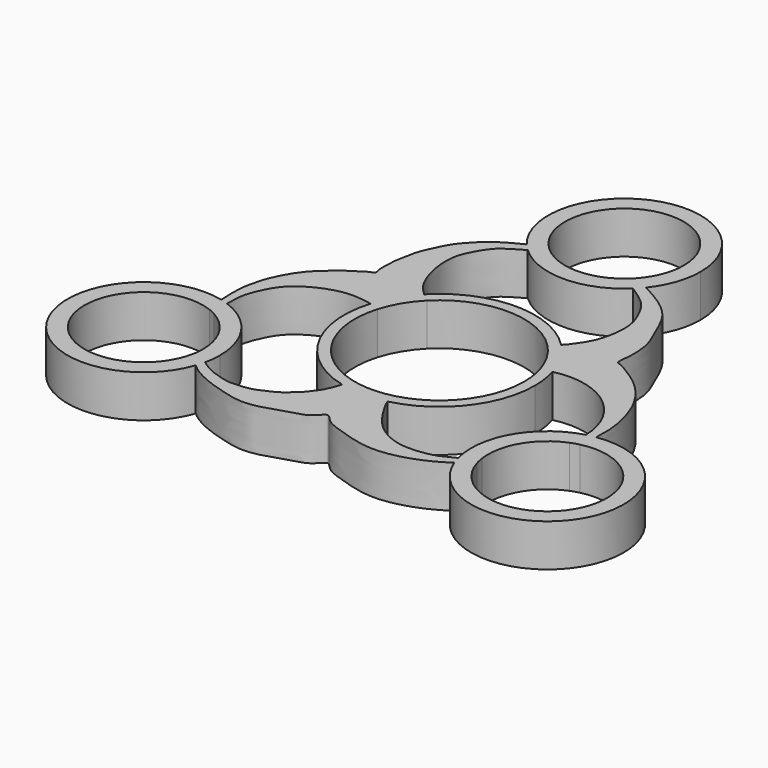
from build123d import *

# Parameters (mm, degrees)
F1_DEPTH = 6.35


with BuildPart() as f1:
    # F0 (on Top) → F1 (new body)
    with BuildSketch(Plane.XY):
        with BuildLine():
            ThreePointArc((12.1979827597, 3.535423114), (12.5738693537, 1.7854437757), (12.7, 0))
            ThreePointArc((12.7, 0), (10.0261967093, -7.79521517), (3.1306488904, -12.3080882969))
            add(Edge.make_bspline(
                [(3.363740595, -13.9083727332), (3.2442211047, -13.5834802382), (3.0616730097, -12.9484213085), (3.1089422782, -12.5172223169), (3.1306488904, -12.3080882969)],
                knots=[0.9737577336, 0.9737577336, 0.9737577336, 0.9737577336, 0.9873943893, 1, 1, 1, 1], degree=3))
            ThreePointArc((3.363740595, -13.9083727332), (11.2447884463, -8.8494245957), (14.309352986, 0))
            ThreePointArc((14.309352986, 0), (14.1647786053, 2.0289479883), (13.7339768745, 4.016897072))
            ThreePointArc((13.7339768745, 4.016897072), (12.9568547986, 3.8052706492), (12.1979827597, 3.535423114))
        make_face()
        with BuildLine():
            ThreePointArc((9.0393838541, 8.9207364908), (10.954763129, 6.4251976457), (12.1979827597, 3.535423114))
            ThreePointArc((12.1979827597, 3.535423114), (12.9568547986, 3.8052706492), (13.7339768745, 4.016897072))
            ThreePointArc((13.7339768745, 4.016897072), (12.356609853, 7.2160775923), (10.2471131468, 9.9877051935))
            add(Edge.make_bspline(
                [(10.2471131468, 9.9877051935), (9.9232107522, 9.6798780377), (9.351132595, 9.2068135599), (9.1315325532, 9.0053976698), (9.0393838541, 8.9207364908)],
                knots=[0.9630977835, 0.9630977835, 0.9630977835, 0.9630977835, 0.9846295847, 1, 1, 1, 1], degree=3))
        make_face()
        with BuildLine():
            add(Edge.make_bspline(
                [(3.363740595, -13.9083727332), (3.2442211047, -13.5834802382), (3.0616730097, -12.9484213085), (3.1089422782, -12.5172223169), (3.1306488904, -12.3080882969)],
                knots=[0.9737577336, 0.9737577336, 0.9737577336, 0.9737577336, 0.9873943893, 1, 1, 1, 1], degree=3))
            ThreePointArc((3.1306488904, -12.3080882969), (-0.0390202402, -12.6999400558), (-3.2062216412, -12.2886184247))
            add(Edge.make_bspline(
                [(-3.2062216412, -12.2886184247), (-3.2435862999, -12.7247349168), (-3.2885775207, -13.2545873407), (-3.4299574494, -13.7893304451), (-3.4577927192, -13.8852890639)],
                knots=[0, 0, 0, 0, 0.0176926318, 0.0215554453, 0.0215554453, 0.0215554453, 0.0215554453], degree=3))
            ThreePointArc((-3.4577927192, -13.8852890639), (-0.0484217354, -14.309271058), (3.363740595, -13.9083727332))
        make_face()
        with BuildLine():
            ThreePointArc((-9.0313311184, 8.9288889695), (0.005729517, 12.6999987076), (9.0393838541, 8.9207364908))
            add(Edge.make_bspline(
                [(10.2471131468, 9.9877051935), (9.9232107522, 9.6798780377), (9.351132595, 9.2068135599), (9.1315325532, 9.0053976698), (9.0393838541, 8.9207364908)],
                knots=[0.9630977835, 0.9630977835, 0.9630977835, 0.9630977835, 0.9846295847, 1, 1, 1, 1], degree=3))
            ThreePointArc((10.2471131468, 9.9877051935), (-0.0109633608, 14.3093487861), (-10.2624056216, 9.9719914628))
            add(Edge.make_bspline(
                [(-9.0313311184, 8.9288889695), (-9.4487098634, 9.2705061134), (-9.8662421937, 9.6122685884), (-10.2624056216, 9.9719914628)],
                knots=[0, 0, 0, 0, 0.0111174301, 0.0111174301, 0.0111174301, 0.0111174301], degree=3))
        make_face()
        with BuildLine():
            ThreePointArc((10.2471131468, 9.9877051935), (12.356609853, 7.2160775923), (13.7339768745, 4.016897072))
            ThreePointArc((13.7339768745, 4.016897072), (22.6213268762, 2.0857346054), (26.7638742582, -6.0107880872))
            ThreePointArc((26.7638742582, -6.0107880872), (27.4125460464, -5.8521775606), (28.0693734163, -5.7317192929))
            add(Edge.make_bspline(
                [(28.0693734163, -5.7317192928), (28.0908448663, -5.3731517648), (28.1861747627, -3.0109562541), (27.749558093, -0.5133237083), (26.6719185003, 2.9301219991), (25.4157041022, 4.8818668184), (25.0606077232, 5.4096449257), (23.1974632753, 7.8967221343), (18.7843205423, 10.5309990469), (18.0312497954, 10.5798070842), (18.3811975836, 12.6295870836), (18.335387886, 16.2496050809), (16.6672868668, 19.632117318), (15.0493924505, 23.6629486703), (11.9963770049, 25.9005801835), (9.3079958484, 27.3351514106), (8.9392781783, 27.5237386375)],
                knots=[0.0686911974, 0.0686911974, 0.0686911974, 0.0686911974, 0.0770625743, 0.1250692546, 0.1682015773, 0.2016986428, 0.2192050888, 0.2596345178, 0.3116854663, 0.3277616325, 0.357626719, 0.4018708944, 0.4463436454, 0.4924730526, 0.5489378858, 0.5577650476, 0.5577650476, 0.5577650476, 0.5577650476], degree=3))
            ThreePointArc((8.9392781783, 27.5237386375), (8.4361841281, 26.9344845866), (7.8943251244, 26.3806680284))
            add(Edge.make_bspline(
                [(7.8943251244, 26.3806680284), (8.4148020655, 26.072489779), (9.8207087272, 25.0972655112), (11.4008317967, 23.8393962796), (12.7154437587, 21.3058333832), (13.4643703621, 19.2153114545), (13.487767982, 16.5541309423), (12.7738805207, 13.4867000838), (11.6527838604, 11.777088674), (10.936534424, 10.6698737269), (10.366109532, 10.1007958017), (10.2471131468, 9.9877051935)],
                knots=[0.6848165544, 0.6848165544, 0.6848165544, 0.6848165544, 0.7057956752, 0.7426414418, 0.7804706255, 0.8144755937, 0.8516859329, 0.8922387418, 0.9247476761, 0.9551873556, 0.9630977835, 0.9630977835, 0.9630977835, 0.9630977835], degree=3))
        make_face()
        with BuildLine():
            add(Edge.make_bspline(
                [(-3.2062216412, -12.2886184247), (-3.2435862999, -12.7247349168), (-3.2885775207, -13.2545873407), (-3.4299574494, -13.7893304451), (-3.4577927192, -13.8852890639)],
                knots=[0, 0, 0, 0, 0.0176926318, 0.0215554453, 0.0215554453, 0.0215554453, 0.0215554453], degree=3))
            ThreePointArc((-3.2062216412, -12.2886184247), (-11.0679306792, -6.228234941), (-12.1680586093, 3.6370798286))
            add(Edge.make_bspline(
                [(-13.6805620316, 4.1952121968), (-13.4436838321, 4.1415517594), (-12.7953614065, 3.9690441824), (-12.4205580368, 3.769996542), (-12.1680586093, 3.6370798286)],
                knots=[0.9804169862, 0.9804169862, 0.9804169862, 0.9804169862, 0.9869875731, 1, 1, 1, 1], degree=3))
            ThreePointArc((-13.6805620316, 4.1952121968), (-12.4562005584, -7.0427729288), (-3.4577927192, -13.8852890639))
        make_face()
        with BuildLine():
            add(Edge.make_bspline(
                [(18.7441266975, -19.9228869496), (18.0486010574, -20.282431647), (16.5041031929, -21.1337661556), (14.3497934766, -21.5215057085), (11.2348222617, -21.7472578966), (7.8237393097, -20.2593616193), (5.6360308604, -18.0063979855), (4.1304020556, -15.5442912857), (3.5977305956, -14.5157527694), (3.3928512144, -13.9875047789), (3.363740595, -13.9083727332)],
                knots=[0.7955891005, 0.7955891005, 0.7955891005, 0.7955891005, 0.8189494254, 0.841960922, 0.8688237268, 0.8981267776, 0.9256229436, 0.9515003665, 0.9704363381, 0.9737577336, 0.9737577336, 0.9737577336, 0.9737577336], degree=3))
            ThreePointArc((3.363740595, -13.9083727332), (-0.0484217354, -14.309271058), (-3.4577927192, -13.8852890639))
            add(Edge.make_bspline(
                [(-3.4577927192, -13.8852890639), (-3.56467622, -14.2537565951), (-3.8875885257, -15.0858670187), (-4.395377985, -16.3369768283), (-5.1592727376, -17.2342121704), (-5.8768462607, -18.2950992181), (-6.9156654614, -19.1057392203), (-7.9469878233, -20.0471955678), (-9.1177528934, -20.5439332885), (-10.4408920068, -21.2379911781), (-11.9275421158, -21.5685916523), (-13.3895555039, -21.6459776552), (-13.8617944711, -21.6400506083), (-14.3017979669, -21.7027035652), (-17.183723559, -21.0200808639), (-18.7684540581, -20.0590219662), (-19.5179344331, -19.4775341217)],
                knots=[0.0215554453, 0.0215554453, 0.0215554453, 0.0215554453, 0.0363881028, 0.0548777285, 0.0715243999, 0.0887731028, 0.1064890588, 0.1245483308, 0.1418573875, 0.1605160383, 0.179942663, 0.1984165029, 0.2084162614, 0.2180022527, 0.2438992002, 0.2696875695, 0.2696875695, 0.2696875695, 0.2696875695], degree=3))
            ThreePointArc((-19.5179344331, -19.4775341217), (-19.6842633145, -20.140683936), (-19.8899435093, -20.7927028242))
            add(Edge.make_bspline(
                [(-19.8899435093, -20.7927028242), (-19.5053999908, -21.1412232423), (-18.421181972, -21.9802458066), (-16.0493936535, -23.1187044109), (-14.0030480662, -23.7091152957), (-9.4186989056, -25.2065289459), (-4.4872481249, -23.2076928696), (-1.3008667338, -22.5759404404), (-0.0119091358, -20.3631569563), (1.1345603492, -22.2720709759), (3.8195402322, -23.1392079338), (7.6272449858, -24.42130256), (11.7818612833, -24.4535976361), (16.3095086913, -22.95262019), (18.294497797, -21.702246116), (19.1372684615, -21.1419244632)],
                knots=[0.3583161785, 0.3583161785, 0.3583161785, 0.3583161785, 0.3741552252, 0.4000090879, 0.4227597006, 0.4556567182, 0.4912178975, 0.5190290749, 0.5393412725, 0.5581268934, 0.5841470097, 0.6149491691, 0.6463952944, 0.6807440143, 0.7044884009, 0.7044884009, 0.7044884009, 0.7044884009], degree=3))
            ThreePointArc((19.1372684615, -21.1419244632), (18.9236082439, -20.5379170475), (18.7441266975, -19.9228869496))
        make_face()
        with BuildLine():
            ThreePointArc((-12.1680586093, 3.6370798286), (-10.9249412906, 6.475774687), (-9.0313311184, 8.9288889695))
            add(Edge.make_bspline(
                [(-9.0313311184, 8.9288889695), (-9.4487098634, 9.2705061134), (-9.8662421937, 9.6122685884), (-10.2624056216, 9.9719914628)],
                knots=[0, 0, 0, 0, 0.0111174301, 0.0111174301, 0.0111174301, 0.0111174301], degree=3))
            ThreePointArc((-10.2624056216, 9.9719914628), (-12.3149997841, 7.2868623696), (-13.6805620316, 4.1952121968))
            add(Edge.make_bspline(
                [(-13.6805620316, 4.1952121968), (-13.4436838321, 4.1415517594), (-12.7953614065, 3.9690441824), (-12.4205580368, 3.769996542), (-12.1680586093, 3.6370798286)],
                knots=[0.9804169862, 0.9804169862, 0.9804169862, 0.9804169862, 0.9869875731, 1, 1, 1, 1], degree=3))
        make_face()
        with BuildLine():
            ThreePointArc((28.0693734163, -5.7317192929), (27.4125460464, -5.8521775606), (26.7638742582, -6.0107880872))
            ThreePointArc((26.7638742582, -6.0107880872), (26.7154514397, -7.4054133304), (26.4847933941, -8.7816840901))
            ThreePointArc((26.4847933941, -8.7816840901), (27.1211091404, -8.5534785531), (27.7729255559, -8.3742835288))
            add(Edge.make_bspline(
                [(27.7729255559, -8.3742835288), (27.9153636471, -7.5821879417), (28.0154450564, -6.6323086159), (28.0693734163, -5.7317192928)],
                knots=[0.0476653874, 0.0476653874, 0.0476653874, 0.0476653874, 0.0686911974, 0.0686911974, 0.0686911974, 0.0686911974], degree=3))
        make_face()
        with BuildLine():
            ThreePointArc((26.4847933941, -8.7816840901), (26.7154514397, -7.4054133304), (26.7638742582, -6.0107880872))
            ThreePointArc((26.7638742582, -6.0107880872), (19.8993963954, -11.3212767476), (18.7441266975, -19.9228869496))
            add(Edge.make_bspline(
                [(21.0074985339, -18.3299627331), (20.8758294418, -18.4776732411), (20.2330176684, -19.2024066572), (19.4784607209, -19.5448948869), (18.7861304092, -19.9011735706), (18.7441266975, -19.9228869496)],
                knots=[0.7662125489, 0.7662125489, 0.7662125489, 0.7662125489, 0.7721682582, 0.7941783396, 0.7955891005, 0.7955891005, 0.7955891005, 0.7955891005], degree=3))
            ThreePointArc((21.0074985339, -18.3299627331), (22.0905705657, -12.6061156205), (26.4847933941, -8.7816840901))
        make_face()
        with BuildLine():
            add(Edge.make_bspline(
                [(21.0074985339, -18.3299627331), (20.8758294418, -18.4776732411), (20.2330176684, -19.2024066572), (19.4784607209, -19.5448948869), (18.7861304092, -19.9011735706), (18.7441266975, -19.9228869496)],
                knots=[0.7662125489, 0.7662125489, 0.7662125489, 0.7662125489, 0.7721682582, 0.7941783396, 0.7955891005, 0.7955891005, 0.7955891005, 0.7955891005], degree=3))
            ThreePointArc((18.7441266975, -19.9228869496), (18.9236082439, -20.5379170475), (19.1372684615, -21.1419244632))
            add(Edge.make_bspline(
                [(19.1372684615, -21.1419244632), (19.375504243, -20.9835318275), (20.0960831119, -20.4976698432), (20.8777393147, -19.9759281537), (21.2980232313, -19.6212498212)],
                knots=[0.7044884009, 0.7044884009, 0.7044884009, 0.7044884009, 0.7112005027, 0.7245782298, 0.7245782298, 0.7245782298, 0.7245782298], degree=3))
            ThreePointArc((21.2980232313, -19.6212498212), (21.1286962311, -18.9810205461), (21.0074985339, -18.3299627331))
        make_face()
        with BuildLine():
            ThreePointArc((-13.6805620316, 4.1952121968), (-12.3149997841, 7.2868623696), (-10.2624056216, 9.9719914628))
            add(Edge.make_bspline(
                [(-10.2624056216, 9.9719914628), (-10.7762356065, 10.4385574962), (-12.0701262188, 11.7836146151), (-13.1133522735, 14.5988264438), (-13.5488715258, 16.8425720746), (-13.6112462054, 19.6390222529), (-12.6179615134, 21.8826004391), (-11.2252292617, 24.1374130376), (-9.9097624261, 25.0601310132), (-8.4142072138, 25.9632491001), (-7.8031976483, 26.2945871618)],
                knots=[0.0111174301, 0.0111174301, 0.0111174301, 0.0111174301, 0.0255369058, 0.0501589029, 0.0704799639, 0.0922653526, 0.1133436415, 0.1345486053, 0.1523387172, 0.1705841628, 0.1705841628, 0.1705841628, 0.1705841628], degree=3))
            ThreePointArc((-7.8031976483, 26.2945871618), (-8.3174588735, 26.8065858605), (-8.7981938428, 27.3501860486))
            add(Edge.make_bspline(
                [(-8.7981938428, 27.3501860486), (-9.3008746077, 27.1141698538), (-10.2648697648, 26.631366973), (-11.2205700524, 26.0765871705), (-12.5077872547, 25.2419913168), (-13.5878297754, 24.2642475313), (-14.8266948114, 22.9775900037), (-15.7640079059, 21.7857963953), (-16.3601601941, 20.5369041311), (-17.0170024392, 19.2950238203), (-17.6605076418, 17.6054504392), (-17.7666020566, 16.8660360184), (-17.9689277925, 15.8439929239), (-18.2780826486, 14.5541624619), (-18.3309003318, 12.8876446559), (-18.3467578229, 11.5218615298), (-17.9795074421, 10.6008301963), (-18.9501500085, 10.4173362769), (-19.6024758542, 9.85743987), (-20.7203525072, 9.2646019513), (-22.1224625096, 8.1909741441), (-23.6705510338, 6.8483154141), (-24.6220525536, 5.8773240915), (-25.4499207491, 4.7537323699), (-26.2162314301, 3.5206531279), (-26.8908201735, 2.0300349867), (-27.2712398353, 1.1575955517), (-27.7898644912, -0.8805960027), (-28.0072247707, -2.066957359), (-28.0597819575, -3.9941490782), (-27.9650258271, -5.6406480469), (-27.9447560089, -5.9324288341)],
                knots=[0.272936701, 0.272936701, 0.272936701, 0.272936701, 0.2887777021, 0.3031918976, 0.319418999, 0.3356933449, 0.3534827997, 0.3699338291, 0.3853607611, 0.4015194954, 0.4192285536, 0.4307941219, 0.4440313196, 0.4595101079, 0.4768532228, 0.4927431634, 0.504260623, 0.5158482459, 0.5283617488, 0.5431378455, 0.5610783945, 0.5802108476, 0.5957692543, 0.6112674735, 0.627599259, 0.6443127052, 0.6577531603, 0.676599654, 0.6913368875, 0.7144941722, 0.7197456255, 0.7197456255, 0.7197456255, 0.7197456255], degree=3))
            ThreePointArc((-27.9447560089, -5.9324288341), (-27.367786238, -6.0909132425), (-26.7999005537, -6.2793735135))
            add(Edge.make_bspline(
                [(-26.7999005537, -6.2793735135), (-26.8048058193, -5.9710391039), (-26.8002842833, -5.0183376748), (-26.6902560699, -3.3465727044), (-25.8799280703, -1.2809508318), (-24.4697637739, 1.4971779335), (-21.1641836673, 3.6006813244), (-17.9496805149, 4.6242605842), (-15.6583644342, 4.5471697783), (-14.1750226558, 4.3072232365), (-13.6805620316, 4.1952121968)],
                knots=[0.8240259196, 0.8240259196, 0.8240259196, 0.8240259196, 0.8330622341, 0.8517096932, 0.8714224213, 0.8946727522, 0.9209129012, 0.9452655147, 0.9667015134, 0.9804169862, 0.9804169862, 0.9804169862, 0.9804169862], degree=3))
        make_face()
        with BuildLine():
            ThreePointArc((-7.8031976483, 26.2945871618), (0.0626780115, 23.2167052828), (7.8943251244, 26.3806680284))
            add(Edge.make_bspline(
                [(5.0609472835, 27.3377091334), (5.4064251806, 27.2499397098), (6.293948707, 27.2199440502), (7.3427878567, 26.7072373271), (7.8943251244, 26.3806680284)],
                knots=[0.6434177254, 0.6434177254, 0.6434177254, 0.6434177254, 0.6625854696, 0.6848165544, 0.6848165544, 0.6848165544, 0.6848165544], degree=3))
            ThreePointArc((5.0609472835, 27.3377091334), (0.0211748238, 25.7565586475), (-5.0260726198, 27.3136830957))
            add(Edge.make_bspline(
                [(-7.8031976483, 26.2945871618), (-7.6884792357, 26.356796624), (-7.0896108618, 26.6725649375), (-6.4348697652, 26.9157154858), (-5.3178085882, 27.1302396322), (-5.0260726198, 27.3136830957)],
                knots=[0.1705841628, 0.1705841628, 0.1705841628, 0.1705841628, 0.174009786, 0.189308331, 0.2026657268, 0.2026657268, 0.2026657268, 0.2026657268], degree=3))
        make_face()
        with BuildLine():
            add(Edge.make_bspline(
                [(5.0609472835, 27.3377091334), (5.4064251806, 27.2499397098), (6.293948707, 27.2199440502), (7.3427878567, 26.7072373271), (7.8943251244, 26.3806680284)],
                knots=[0.6434177254, 0.6434177254, 0.6434177254, 0.6434177254, 0.6625854696, 0.6848165544, 0.6848165544, 0.6848165544, 0.6848165544], degree=3))
            ThreePointArc((7.8943251244, 26.3806680284), (8.4361841281, 26.9344845866), (8.9392781783, 27.5237386375))
            add(Edge.make_bspline(
                [(8.9392781783, 27.5237386375), (8.1220241857, 27.9417377645), (7.27892146, 28.3334051291), (6.5316696861, 28.6158293985)],
                knots=[0.5577650476, 0.5577650476, 0.5577650476, 0.5577650476, 0.5773302432, 0.5773302432, 0.5773302432, 0.5773302432], degree=3))
            ThreePointArc((6.5316696861, 28.6158293985), (5.8314312055, 27.9363538422), (5.0609472835, 27.3377091334))
        make_face()
        with BuildLine():
            ThreePointArc((41.2318883914, -17.029652372), (37.2464251075, -8.3564884117), (28.0693734163, -5.7317192929))
            add(Edge.make_bspline(
                [(27.7729255559, -8.3742835288), (27.9153636471, -7.5821879417), (28.0154450564, -6.6323086159), (28.0693734163, -5.7317192928)],
                knots=[0.0476653874, 0.0476653874, 0.0476653874, 0.0476653874, 0.0686911974, 0.0686911974, 0.0686911974, 0.0686911974], degree=3))
            ThreePointArc((27.7729255559, -8.3742835288), (35.3243253712, -10.0629609188), (38.6918883914, -17.029652372))
            ThreePointArc((38.6918883914, -17.029652372), (31.1119911978, -25.8225887778), (21.2980232313, -19.6212498212))
            add(Edge.make_bspline(
                [(19.1372684615, -21.1419244632), (19.375504243, -20.9835318275), (20.0960831119, -20.4976698432), (20.8777393147, -19.9759281537), (21.2980232313, -19.6212498212)],
                knots=[0.7044884009, 0.7044884009, 0.7044884009, 0.7044884009, 0.7112005027, 0.7245782298, 0.7245782298, 0.7245782298, 0.7245782298], degree=3))
            ThreePointArc((19.1372684615, -21.1419244632), (31.8933345659, -28.2666783531), (41.2318883914, -17.029652372))
        make_face()
        with BuildLine():
            ThreePointArc((-19.8899435093, -20.7927028242), (-19.6842633145, -20.140683936), (-19.5179344331, -19.4775341217))
            add(Edge.make_bspline(
                [(-19.5179344331, -19.4775341217), (-19.5480873984, -19.4541398029), (-20.2385646864, -18.9134540134), (-21.2032781619, -17.9973679304), (-21.6108542907, -17.7847042589), (-21.8079642143, -17.8525900961), (-21.8318301495, -17.8624673324)],
                knots=[0.2696875695, 0.2696875695, 0.2696875695, 0.2696875695, 0.2707250827, 0.2934984271, 0.3044311145, 0.3059181156, 0.3059181156, 0.3059181156, 0.3059181156], degree=3))
            ThreePointArc((-21.8318301495, -17.8624673324), (-21.8768443076, -18.2496468629), (-21.9387872394, -18.6344810304))
            add(Edge.make_bspline(
                [(-21.9387872394, -18.6344810304), (-21.9075854602, -18.6644968742), (-21.4991423455, -19.0559305442), (-20.784352374, -19.9304787362), (-20.0819727379, -20.6186624261), (-19.8899435093, -20.7927028242)],
                knots=[0.3263959289, 0.3263959289, 0.3263959289, 0.3263959289, 0.3283204128, 0.3504066447, 0.3583161785, 0.3583161785, 0.3583161785, 0.3583161785], degree=3))
        make_face()
        with BuildLine():
            add(Edge.make_bspline(
                [(-19.5179344331, -19.4775341217), (-19.5480873984, -19.4541398029), (-20.2385646864, -18.9134540134), (-21.2032781619, -17.9973679304), (-21.6108542907, -17.7847042589), (-21.8079642143, -17.8525900961), (-21.8318301495, -17.8624673324)],
                knots=[0.2696875695, 0.2696875695, 0.2696875695, 0.2696875695, 0.2707250827, 0.2934984271, 0.3044311145, 0.3059181156, 0.3059181156, 0.3059181156, 0.3059181156], degree=3))
            ThreePointArc((-19.5179344331, -19.4775341217), (-19.319228377, -18.2607551016), (-19.2527351451, -17.029652372))
            ThreePointArc((-19.2527351451, -17.029652372), (-21.3279048586, -10.4621528242), (-26.7999005537, -6.2793735135))
            add(Edge.make_bspline(
                [(-26.4177782054, -9.229508636), (-26.4493307908, -9.0976381199), (-26.6579238649, -8.5139773475), (-26.762165792, -7.4727064796), (-26.7949329577, -6.5916258799), (-26.7999005537, -6.2793735135)],
                knots=[0.7924239305, 0.7924239305, 0.7924239305, 0.7924239305, 0.7979784643, 0.814874782, 0.8240259196, 0.8240259196, 0.8240259196, 0.8240259196], degree=3))
            ThreePointArc((-26.4177782054, -9.229508636), (-23.0359198866, -12.495524407), (-21.7927351451, -17.029652372))
            ThreePointArc((-21.7927351451, -17.029652372), (-21.8025142748, -17.4465184109), (-21.8318301495, -17.8624673324))
        make_face()
        with BuildLine():
            ThreePointArc((-8.7981938428, 27.3501860486), (-8.3174588735, 26.8065858605), (-7.8031976483, 26.2945871618))
            add(Edge.make_bspline(
                [(-7.8031976483, 26.2945871618), (-7.6884792357, 26.356796624), (-7.0896108618, 26.6725649375), (-6.4348697652, 26.9157154858), (-5.3178085882, 27.1302396322), (-5.0260726198, 27.3136830957)],
                knots=[0.1705841628, 0.1705841628, 0.1705841628, 0.1705841628, 0.174009786, 0.189308331, 0.2026657268, 0.2026657268, 0.2026657268, 0.2026657268], degree=3))
            ThreePointArc((-5.0260726198, 27.3136830957), (-5.6525353954, 27.7849779497), (-6.2350425653, 28.3096300684))
            add(Edge.make_bspline(
                [(-6.2350425653, 28.3096300684), (-6.4996721533, 28.2447514426), (-7.2352724841, 28.041030397), (-8.1163824284, 27.6678086077), (-8.7335223956, 27.3805502677), (-8.7981938428, 27.3501860486)],
                knots=[0.2441441164, 0.2441441164, 0.2441441164, 0.2441441164, 0.2534785462, 0.2708987068, 0.272936701, 0.272936701, 0.272936701, 0.272936701], degree=3))
        make_face()
        with BuildLine():
            add(Edge.make_bspline(
                [(8.9392781783, 27.5237386375), (8.1220241857, 27.9417377645), (7.27892146, 28.3334051291), (6.5316696861, 28.6158293985)],
                knots=[0.5577650476, 0.5577650476, 0.5577650476, 0.5577650476, 0.5773302432, 0.5773302432, 0.5773302432, 0.5773302432], degree=3))
            ThreePointArc((8.9392781783, 27.5237386375), (10.789366283, 30.8736730809), (11.43, 34.6465334296))
            ThreePointArc((11.43, 34.6465334296), (-3.8782434411, 45.3984694326), (-8.7981938428, 27.3501860486))
            add(Edge.make_bspline(
                [(-6.2350425653, 28.3096300684), (-6.4996721533, 28.2447514426), (-7.2352724841, 28.041030397), (-8.1163824284, 27.6678086077), (-8.7335223956, 27.3805502677), (-8.7981938428, 27.3501860486)],
                knots=[0.2441441164, 0.2441441164, 0.2441441164, 0.2441441164, 0.2534785462, 0.2708987068, 0.272936701, 0.272936701, 0.272936701, 0.272936701], degree=3))
            ThreePointArc((-6.2350425653, 28.3096300684), (-3.4352999574, 42.8459733009), (8.89, 34.6465334296))
            ThreePointArc((8.89, 34.6465334296), (8.2794517786, 31.4088215454), (6.5316696861, 28.6158293985))
        make_face()
        with BuildLine():
            add(Edge.make_bspline(
                [(-26.4177782054, -9.229508636), (-26.4493307908, -9.0976381199), (-26.6579238649, -8.5139773475), (-26.762165792, -7.4727064796), (-26.7949329577, -6.5916258799), (-26.7999005537, -6.2793735135)],
                knots=[0.7924239305, 0.7924239305, 0.7924239305, 0.7924239305, 0.7979784643, 0.814874782, 0.8240259196, 0.8240259196, 0.8240259196, 0.8240259196], degree=3))
            ThreePointArc((-26.7999005537, -6.2793735135), (-27.367786238, -6.0909132425), (-27.9447560089, -5.9324288341))
            add(Edge.make_bspline(
                [(-27.9447560089, -5.9324288341), (-27.8836843278, -6.8115459044), (-27.7733376394, -7.7922095292), (-27.6438520179, -7.1954960472), (-27.6492873184, -8.1133057892), (-27.4940984055, -8.671519699), (-27.4727678432, -8.7394044915)],
                knots=[0.7197456255, 0.7197456255, 0.7197456255, 0.7197456255, 0.7355679222, 0.7400306535, 0.7540739268, 0.7561027786, 0.7561027786, 0.7561027786, 0.7561027786], degree=3))
            ThreePointArc((-27.4727678432, -8.7394044915), (-26.9372480443, -8.9671821316), (-26.4177782054, -9.229508636))
        make_face()
        with BuildLine():
            ThreePointArc((-27.9447560089, -5.9324288341), (-40.7314850766, -22.4764426942), (-19.8899435093, -20.7927028242))
            add(Edge.make_bspline(
                [(-21.9387872394, -18.6344810304), (-21.9075854602, -18.6644968742), (-21.4991423455, -19.0559305442), (-20.784352374, -19.9304787362), (-20.0819727379, -20.6186624261), (-19.8899435093, -20.7927028242)],
                knots=[0.3263959289, 0.3263959289, 0.3263959289, 0.3263959289, 0.3283204128, 0.3504066447, 0.3583161785, 0.3583161785, 0.3583161785, 0.3583161785], degree=3))
            ThreePointArc((-21.9387872394, -18.6344810304), (-38.4417400507, -21.3690005805), (-27.4727678432, -8.7394044915))
            add(Edge.make_bspline(
                [(-27.9447560089, -5.9324288341), (-27.8836843278, -6.8115459044), (-27.7733376394, -7.7922095292), (-27.6438520179, -7.1954960472), (-27.6492873184, -8.1133057892), (-27.4940984055, -8.671519699), (-27.4727678432, -8.7394044915)],
                knots=[0.7197456255, 0.7197456255, 0.7197456255, 0.7197456255, 0.7355679222, 0.7400306535, 0.7540739268, 0.7561027786, 0.7561027786, 0.7561027786, 0.7561027786], degree=3))
        make_face()
    extrude(amount=F1_DEPTH)


solid = f1.part
